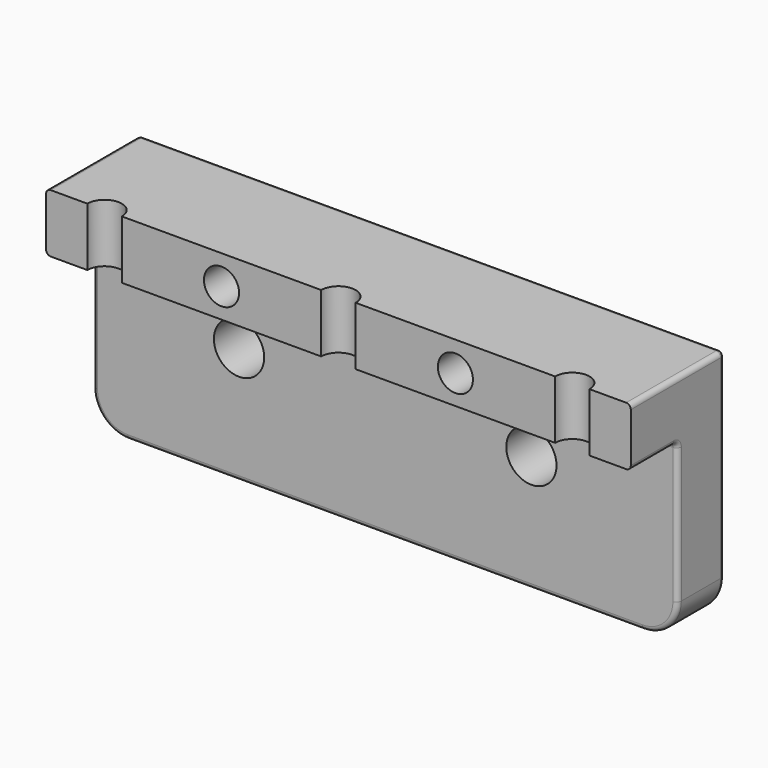
from build123d import *

# Parameters (mm, degrees)
F0_W     = 50
F0_H     = 15
F1_DEPTH = 5
F2_D     = 4.3
F0_H_2   = 5
F3_DEPTH = 10
F5_D     = 2.95
F6_R     = 3
F7_R     = 0.4
F9_D     = 3
F9_DEPTH = 6
F9_TIP   = 0.9012909285


with BuildPart() as f1:
    # F0 (on Front) → F1 (new body)
    with BuildSketch(Plane.XZ):
        with Locations((0, -2.5)):
            Rectangle(F0_W, F0_H)
    extrude(amount=F1_DEPTH)

    # F2 (through all)
    with Locations(Plane(origin=(0, 0, 0), x_dir=(1, 0, 0), z_dir=(0, 1, 0))):
        with Locations((12.5, 0), (-12.5, 0)):
            Hole(F2_D / 2)

    # F0 (on Front) → F3 (join)
    with BuildSketch(Plane.XZ):
        with Locations((0, 7.5)):
            Rectangle(F0_W, F0_H_2)
    extrude(amount=F3_DEPTH)

    # F5 (through all)
    with Locations(Plane.XY.offset(10)):
        with Locations((-20, -10), (0, -10), (20, -10)):
            Hole(F5_D / 2)

    # F6
    f6_edges = [f1.edges().sort_by_distance(p)[0] for p in [
        (-25, -2.5, -10),
        (25, -2.5, -10),
    ]]
    fillet(f6_edges, radius=F6_R)

    # F7
    f7_edges = [f1.edges().sort_by_distance(p)[0] for p in [
        (0, 0, 10),
        (-25, 0, 1.5),
        (-25, -5, 10),
        (25, -5, 10),
        (0, -5, -10),
        (0, -5, 5),
        (25, -5, -1),
        (25, -7.5, 5),
        (25, 0, 1.5),
        (24.12132, -5, -9.12132),
        (-25, -5, -1),
        (-24.12132, -5, -9.12132),
        (24.12132, 0, -9.12132),
        (-25, -7.5, 5),
        (0, 0, -10),
        (-24.12132, 0, -9.12132),
    ]]
    fillet(f7_edges, radius=F7_R)

    # F9
    with Locations(Plane.XZ.offset(10)):
        with Locations((-10, 7.5), (10, 7.4705528095)):
            Hole(F9_D / 2, depth=F9_DEPTH)
            with Locations((0, 0, -(F9_DEPTH + F9_TIP / 2))):  # 118° drill point
                Cone(0, F9_D / 2, F9_TIP, mode=Mode.SUBTRACT)


solid = f1.part
